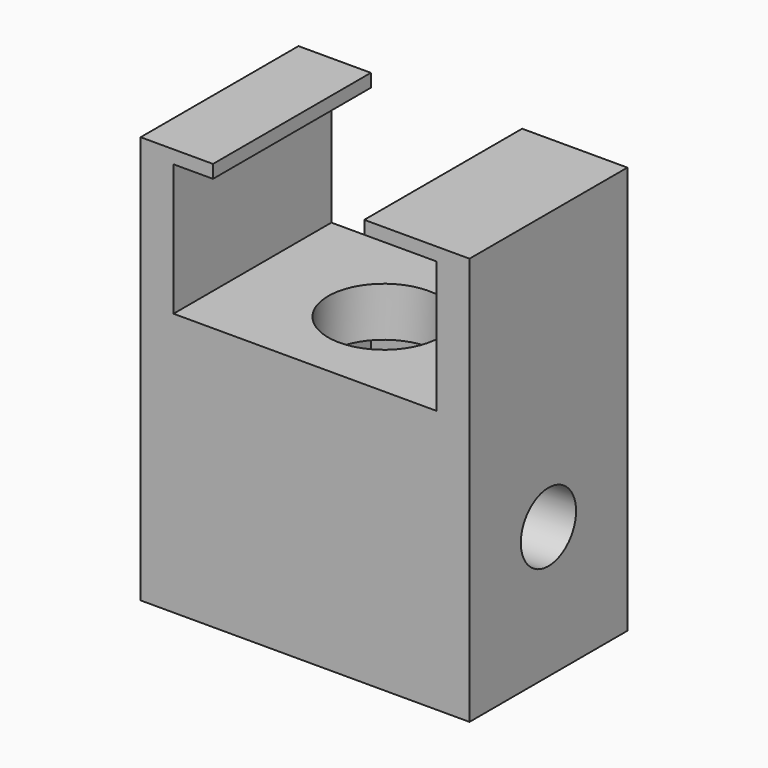
from build123d import *

# Parameters (mm, degrees)
F2_W      = 50
F2_H      = 30
F3_DEPTH  = 30
F0_R      = 8.5
F4_DEPTH  = 20
F5_W      = 5
F5_H      = 30
F6_DEPTH  = 22
F7_W      = 30
F7_H      = 2
F8_DEPTH  = 6
F9_W      = 30
F9_H      = 2
F10_DEPTH = 11
F11_W     = 20
F11_H     = 20
F12_DEPTH = 12.5
F13_W     = 50
F13_H     = 30
F14_DEPTH = 10
F15_DEPTH = 25
F16_R     = 5.25
F17_DEPTH = 50


with BuildPart() as f3:
    # F2 (on offset) → F3 (new body)
    with BuildSketch(Plane.XY.offset(20)):
        Rectangle(F2_W, F2_H)
    extrude(amount=-F3_DEPTH)

    # F0 (on Top) → F4 (cut)
    with BuildSketch(Plane.XY):
        Circle(F0_R)
    extrude(amount=F4_DEPTH, mode=Mode.SUBTRACT)

    # F5 (on face) → F6 (join)
    with BuildSketch(Plane.XY.offset(20)):
        with Locations((-22.5, 0)):
            Rectangle(F5_W, F5_H)
        with Locations((22.5, 0)):
            Rectangle(F5_W, F5_H)
    extrude(amount=F6_DEPTH)

    # F7 (on face) → F8 (join)
    with BuildSketch(Plane.YZ.offset(-20)):
        with Locations((0, 41)):
            Rectangle(F7_W, F7_H)
    extrude(amount=F8_DEPTH)

    # F9 (on face) → F10 (join)
    with BuildSketch(Plane(origin=(20, 0, 0), x_dir=(0, -1, 0), z_dir=(-1, 0, 0))):
        with Locations((0, 41)):
            Rectangle(F9_W, F9_H)
    extrude(amount=F10_DEPTH)

    # F11 (on Top) → F12 (cut, symmetric)
    with BuildSketch(Plane.XY):
        Rectangle(F11_W, F11_H)
    extrude(amount=F12_DEPTH, both=True, mode=Mode.SUBTRACT)

    # F13 (on face) → F14 (join)
    with BuildSketch(Plane(origin=(0, 0, -10), x_dir=(1, 0, 0), z_dir=(0, 0, -1))):
        Rectangle(F13_W, F13_H)
    extrude(amount=F14_DEPTH)

    # F0 (on Top) → F15 (cut)
    with BuildSketch(Plane.XY):
        Circle(F0_R)
    extrude(amount=-F15_DEPTH, mode=Mode.SUBTRACT)

    # F16 (on face) → F17 (cut)
    with BuildSketch(Plane.YZ.offset(25)):
        Circle(F16_R)
    extrude(amount=-F17_DEPTH, mode=Mode.SUBTRACT)


solid = f3.part
